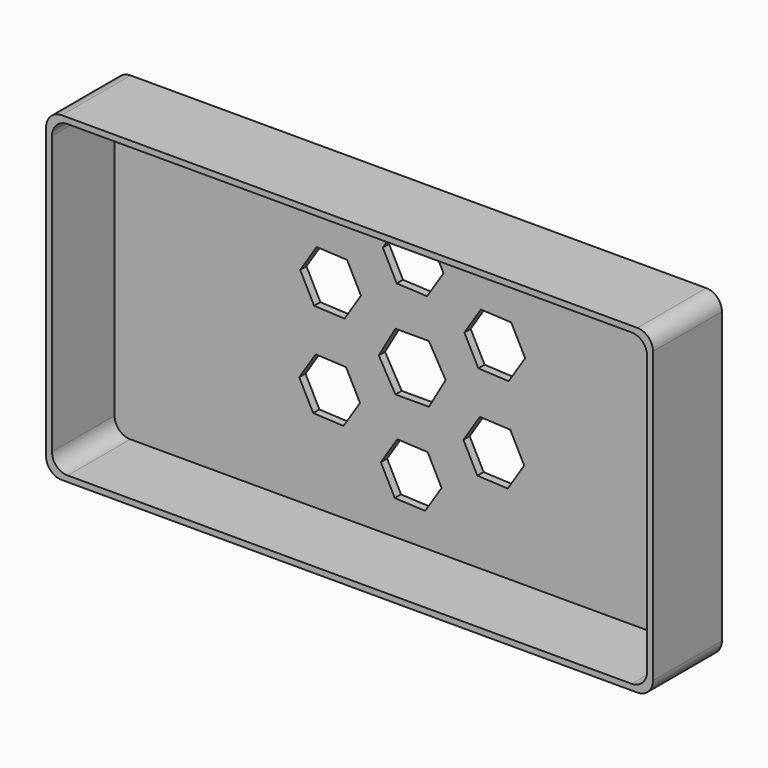
from build123d import *

# Parameters (mm, degrees)
F1_DEPTH = 2
F3_DEPTH = 20
F5_DEPTH = 12.5


# Not quite as in the source:
# - a feature names something its author has since deleted; it is built from what else it names


with BuildPart() as f1:
    # F0 (on Front) → F1 (new body)
    with BuildSketch(Plane.XZ):
        with BuildLine():
            Line((79.8777135909, 45.9989449601), (-67.1222864091, 45.9989449601))
            ThreePointArc((-67.1222864091, 45.9989449601), (-69.9507135339, 44.8273720848), (-71.1222864091, 41.9989449601))
            Line((-71.1222864091, 41.9989449601), (-71.1222864091, -32.0010550399))
            ThreePointArc((-71.1222864091, -32.0010550399), (-69.9507135339, -34.8294821647), (-67.1222864091, -36.0010550399))
            Line((-67.1222864091, -36.0010550399), (79.8777135909, -36.0010550399))
            ThreePointArc((79.8777135909, -36.0010550399), (82.7061407156, -34.8294821647), (83.8777135909, -32.0010550399))
            Line((83.8777135909, -32.0010550399), (83.8777135909, 41.9989449601))
            ThreePointArc((83.8777135909, 41.9989449601), (82.7061407156, 44.8273720848), (79.8777135909, 45.9989449601))
        make_face()
    extrude(amount=F1_DEPTH)

    # F2 (on face) → F3 (join)
    with BuildSketch(Plane.XZ.offset(2)):
        with BuildLine():
            ThreePointArc((83.8777135909, 41.9989449601), (82.7061407156, 44.8273720848), (79.8777135909, 45.9989449601))
            Line((79.8777135909, 45.9989449601), (-67.1222864091, 45.9989449601))
            ThreePointArc((-67.1222864091, 45.9989449601), (-69.9507135339, 44.8273720848), (-71.1222864091, 41.9989449601))
            Line((-71.1222864091, 41.9989449601), (-71.1222864091, -32.0010550399))
            ThreePointArc((-71.1222864091, -32.0010550399), (-69.9507135339, -34.8294821647), (-67.1222864091, -36.0010550399))
            Line((-67.1222864091, -36.0010550399), (79.8777135909, -36.0010550399))
            ThreePointArc((79.8777135909, -36.0010550399), (82.7061407156, -34.8294821647), (83.8777135909, -32.0010550399))
            Line((83.8777135909, -32.0010550399), (83.8777135909, 41.9989449601))
        make_face()
        with BuildLine():
            ThreePointArc((-69.6222864091, 40.4989449601), (-68.4507135339, 43.3273720848), (-65.6222864091, 44.4989449601))
            Line((-65.6222864091, 44.4989449601), (78.3777135909, 44.4989449601))
            ThreePointArc((78.3777135909, 44.4989449601), (81.2061407156, 43.3273720848), (82.3777135909, 40.4989449601))
            Line((82.3777135909, 40.4989449601), (82.3777135909, -30.5010550399))
            ThreePointArc((82.3777135909, -30.5010550399), (81.2061407156, -33.3294821647), (78.3777135909, -34.5010550399))
            Line((78.3777135909, -34.5010550399), (-65.6222864091, -34.5010550399))
            ThreePointArc((-65.6222864091, -34.5010550399), (-68.4507135339, -33.3294821647), (-69.6222864091, -30.5010550399))
            Line((-69.6222864091, -30.5010550399), (-69.6222864091, 40.4989449601))
        make_face(mode=Mode.SUBTRACT)
    extrude(amount=F3_DEPTH)

    # F4 (on face) → F5 (cut, symmetric)
    with BuildSketch(Plane.XZ.offset(2)):
        Polygon((14.3804825891, 28.8355327559), (10.8255747657, 35.7375912952), (3.0707628205, 36.1099800817), (-1.1291413013, 29.5803103289), (2.4257665221, 22.6782517895), (10.1805784673, 22.305863003), align=None)
        Polygon((35.2220927825, 16.5163073577), (31.6671849591, 23.4183658971), (23.9123730139, 23.7907546836), (19.7124688921, 17.2610849307), (23.2673767155, 10.3590263914), (31.0221886607, 9.9866376049), align=None)
        Polygon((30.7742316076, -14.2223389774), (34.9741357295, -7.6926692246), (31.419227906, -0.7906106852), (23.6644159608, -0.4182218987), (19.464511839, -6.9478916516), (23.0194196624, -13.8499501909), align=None)
        Polygon((1.929852416, -25.7397013751), (9.6846643612, -26.1120901616), (13.884568483, -19.5824204088), (10.3296606596, -12.6803618694), (2.5748487144, -12.3079730829), (-1.6250554074, -18.8376428357), align=None)
        Polygon((-22.4666656008, -6.5184174376), (-18.9117577774, -13.420475977), (-11.1569458322, -13.7928647635), (-6.9570417103, -7.2631950106), (-10.5119495338, -0.3611364712), (-18.266761479, 0.0112523153), align=None)
        Polygon((-18.0188044259, 24.2202288976), (-22.2187085477, 17.6905591447), (-18.6638007243, 10.7885006053), (-10.9089887791, 10.4161118188), (-6.7090846573, 16.9457815717), (-10.2639924807, 23.8478401111), align=None)
        Polygon((2.1058970544, -2.4000583217), (10.6495301273, -2.4000583217), (14.9213466637, 4.9989449601), (10.6495301273, 12.3979482418), (2.1058970544, 12.3979482418), (-2.165919482, 4.9989449601), align=None)
    extrude(amount=F5_DEPTH, both=True, mode=Mode.SUBTRACT)


solid = f1.part
